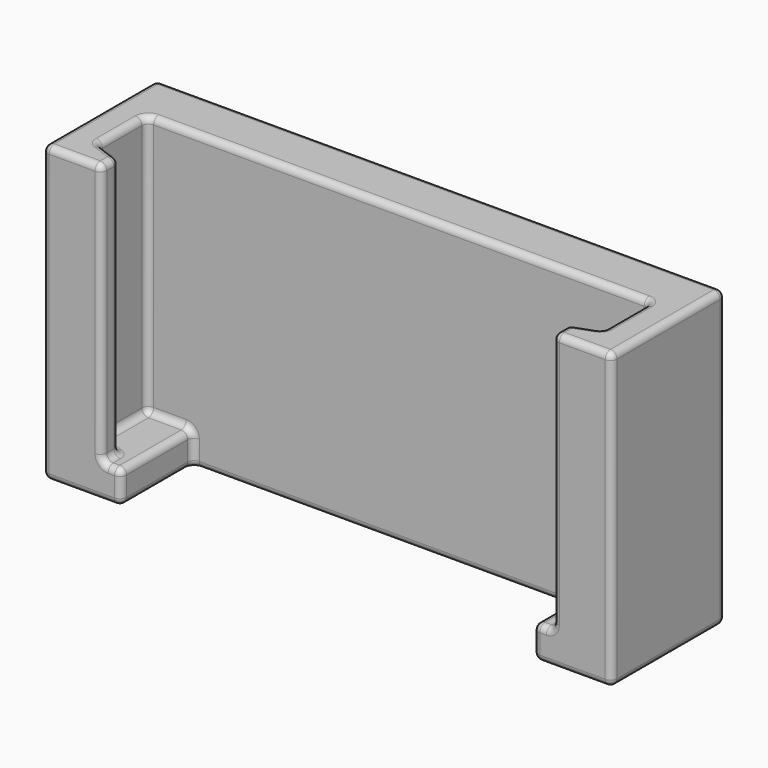
from build123d import *

# Parameters (mm, degrees)
F0_W      = 87
F0_H      = 21.7
F1_DEPTH  = 5
F3_DEPTH  = 40
F5_DEPTH  = 4.6
F6_W      = 2.7
F6_H      = 11.4
F7_DEPTH  = 3.3
F8_W      = 2.7
F8_H      = 11.4
F9_DEPTH  = 3.3
F10_W     = 63
F10_H     = 5
F11_DEPTH = 13.7
F12_R     = 1


with BuildPart() as f1:
    # F0 (on Top) → F1 (new body)
    with BuildSketch(Plane.XY):
        with Locations((43.5, -10.85)):
            Rectangle(F0_W, F0_H)
    extrude(amount=F1_DEPTH)

    # F2 (on face) → F3 (join)
    with BuildSketch(Plane.XY.offset(5)):
        Polygon((87, 0), (0, 0), (0, -21.7), (9, -21.7), (9, -18.6558809371), (5, -17.2), (5, -8), (82, -8), (82, -17.2), (78, -18.6558809371), (78, -21.7), (87, -21.7), align=None)
    extrude(amount=F3_DEPTH)

    # F4 (on face) → F5 (cut)
    with BuildSketch(Plane(origin=(0, 0, 0), x_dir=(-1, 0, 0), z_dir=(0, 1, 0))):
        Polygon((-42.2, 37), (-43.5, 37), (-43.5, 10.6), (-38.9, 10.6), (-38.9, 25.6), (-42.2, 25.6), align=None)
        Polygon((-43.5, 10.6), (-43.5, 37), (-44.8, 37), (-44.8, 25.6), (-48.1, 25.6), (-48.1, 10.6), align=None)
    extrude(amount=-F5_DEPTH, mode=Mode.SUBTRACT)

    # F6 (on face) → F7 (cut)
    with BuildSketch(Plane.YZ.offset(42.2)):
        with Locations((-3.25, 31.3)):
            Rectangle(F6_W, F6_H)
    extrude(amount=-F7_DEPTH, mode=Mode.SUBTRACT)

    # F8 (on face) → F9 (cut)
    with BuildSketch(Plane(origin=(44.8, 0, 0), x_dir=(0, -1, 0), z_dir=(-1, 0, 0))):
        with Locations((3.25, 31.3)):
            Rectangle(F8_W, F8_H)
    extrude(amount=-F9_DEPTH, mode=Mode.SUBTRACT)

    # F10 (on face) → F11 (cut)
    with BuildSketch(Plane.XZ.offset(21.7)):
        with Locations((43.5, 2.5)):
            Rectangle(F10_W, F10_H)
    extrude(amount=-F11_DEPTH, mode=Mode.SUBTRACT)

    # F12
    f12_edges = [f1.edges().sort_by_distance(p)[0] for p in [
        (12, -14.85, 5),
        (12, -14.85, 0),
        (12, -8, 2.5),
        (43.5, -8, 0),
        (5, -8, 25),
        (5, -12.6, 5),
        (9, -18.655881, 25),
        (9, -21.7, 25),
        (10.5, -21.7, 5),
        (9, -20.17794, 5),
        (6, -21.7, 0),
        (0, -21.7, 22.5),
        (43.5, -8, 45),
        (82, -12.6, 45),
        (80, -17.92794, 45),
        (78, -20.17794, 45),
        (82.5, -21.7, 45),
        (87, -10.85, 45),
        (87, -21.7, 22.5),
        (82, -8, 25),
        (78.5, -8, 5),
        (75, -8, 2.5),
        (8.5, -8, 5),
        (78, -21.7, 25),
        (75, -14.85, 5),
        (82, -12.6, 5),
        (76.5, -21.7, 5),
        (78, -20.17794, 5),
        (78, -18.655881, 25),
        (82, -17.2, 25),
        (5, -17.2, 25),
        (4.5, -21.7, 45),
        (9, -20.17794, 45),
        (0, -10.85, 45),
        (43.5, 0, 45),
        (87, 0, 22.5),
        (87, -10.85, 0),
        (81, -21.7, 0),
        (75, -21.7, 2.5),
        (12, -21.7, 2.5),
        (43.5, 0, 0),
        (0, 0, 22.5),
        (0, -10.85, 0),
        (75, -14.85, 0),
        (7, -17.92794, 45),
        (5, -12.6, 45),
        (7, -17.92794, 5),
        (80, -17.92794, 5),
    ]]
    fillet(f12_edges, radius=F12_R)


solid = f1.part
